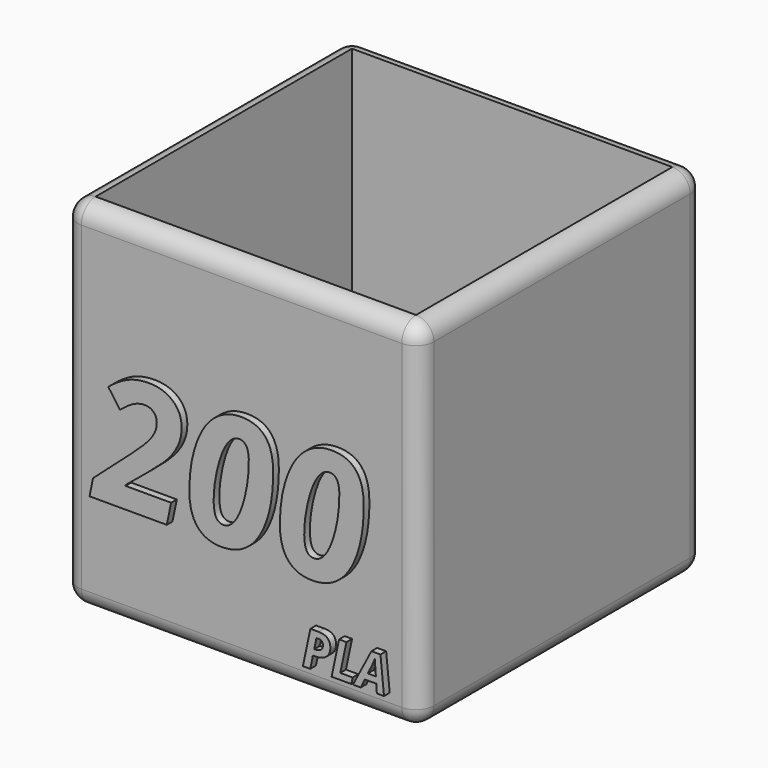
from build123d import *

# Parameters (mm, degrees)
F0_W         = 20
F0_H         = 20
F1_DEPTH     = 20
F2_R         = 1
F3_T         = 1
F4_R         = 0.99999
F7_TEXT_SIZE = 9.2360422116
F8_DEPTH     = 0.4
F9_TEXT_SIZE = 2.7777777778
F10_DEPTH    = 0.4


# Not quite as in the source:
# - a fillet or chamfer is up to 0.001 mm smaller than in the source, because OpenCascade refuses the exact size
# - a shell that OpenCascade refuses in one call is made with other operations: the cavity is built on its own and cut out
# - Text() gives the source's letters only with a copy of the font that has no kerning and outlines rounded to 1/6400 em; it was checked with that copy


with BuildPart() as f1:
    # F0 (on Top) → F1 (new body)
    with BuildSketch(Plane.XY):
        Rectangle(F0_W, F0_H)
    extrude(amount=F1_DEPTH)

    # F2
    f2_edges = [f1.edges().sort_by_distance(p)[0] for p in [
        (10, 10, 10),
        (-10, -10, 10),
        (10, -10, 10),
        (-10, 10, 10),
        (10, 0, 0),
        (0, -10, 0),
        (0, 10, 0),
        (-10, 0, 0),
    ]]
    fillet(f2_edges, radius=F2_R)

    # F3: shell of thickness 1, made by hand


with BuildPart() as f3_core1:
    # F3_t2: copy of F1
    add(f1.part)

    # the walls: a layer under each face that stays
    f3_faces = [f3_core1.faces().sort_by_distance(p)[0] for p in [
        (0, -10, 10.5),
        (-10, 0, 10.5),
        (10, 0, 10.5),
        (0, 10, 10.5),
        (0, 0, 0),
    ]]
    thicken(f3_faces, amount=-F3_T, mode=Mode.SUBTRACT)


with BuildPart() as f1_1:
    add(f1.part)

    # what is left inside the walls is the cavity
    f3_cavity = [f3_core1.part.solids().sort_by_distance(p)[0] for p in [
        (-8.99, 0, 13.666667),
    ]]
    add(f3_cavity, mode=Mode.SUBTRACT)

    # F4 (radius 1 in the source; OpenCascade refuses exactly that, so slightly less here)
    f4_edges = [f1_1.edges().sort_by_distance(p)[0] for p in [
        (9.707107, 9.707107, 20),
        (-9.707107, 9.707107, 20),
        (0, -10, 20),
        (0, 10, 20),
        (-9.707107, -9.707107, 20),
        (10, 0, 20),
        (-10, 0, 20),
        (9.707107, -9.707107, 20),
    ]]
    fillet(f4_edges, radius=F4_R)

    # F7 (on face) → F8 (join)
    with BuildSketch(Plane.XZ.offset(10)):
        with Locations((-8, 6)):
            Text('200', F7_TEXT_SIZE, font='Open Sans', font_style=FontStyle.BOLDITALIC, text_align=(TextAlign.LEFT, TextAlign.BOTTOM))
    extrude(amount=F8_DEPTH)

    # F9 (on face) → F10 (join)
    with BuildSketch(Plane.XZ.offset(10)):
        with Locations((3.6918402778, 1.5)):
            Text('PLA', F9_TEXT_SIZE, font='Open Sans', font_style=FontStyle.BOLDITALIC, text_align=(TextAlign.LEFT, TextAlign.BOTTOM))
    extrude(amount=F10_DEPTH)


solid = f1_1.part
